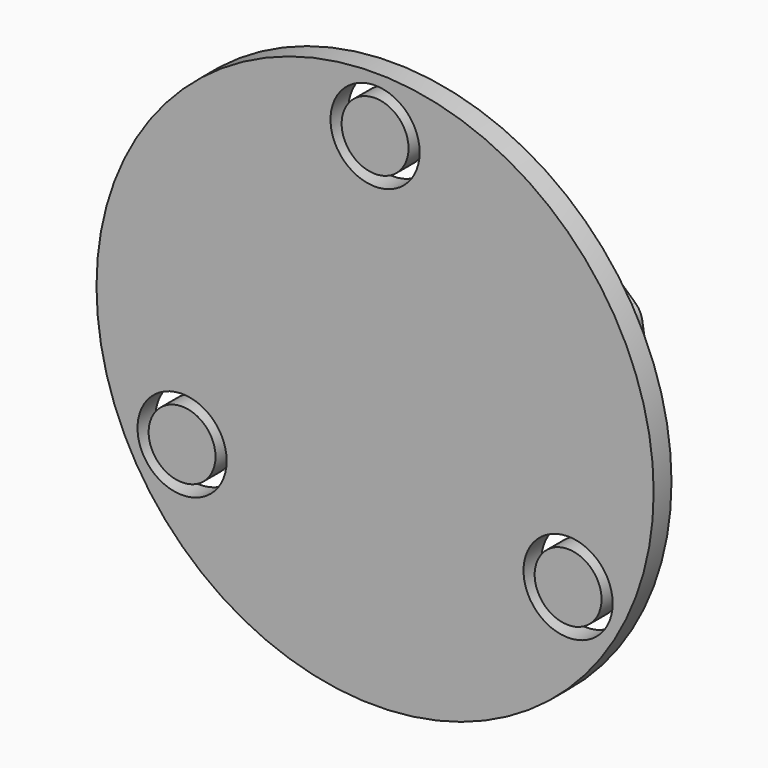
from build123d import *

# Parameters (mm, degrees)
F1_DEPTH      = 13
F2_R          = 1.3
F3_DEPTH      = 5
F4_R          = 1.3
F5_DEPTH      = 25
F6_R          = 1.3
F7_DEPTH      = 5
F8_R          = 25
F9_DEPTH      = 2
F10_R         = 4
F10_R_2       = 3
F11_DEPTH     = 80
F12_T1_DEPTH  = 16.002243982
F12_T3_DEPTH  = 14.8598729542
F12_T5_DEPTH  = 14.7613040686
F12_T7_DEPTH  = 15.2887647241
F12_T9_DEPTH  = 14.7419723435
F12_T11_DEPTH = 14.2482473807


# Not quite as in the source:
# - a fillet or chamfer that OpenCascade refuses, or shapes differently, is made with other operations: its cross-section is extruded or revolved along the edge and cut away or added


with BuildPart() as f1:
    # F0 (on Front) → F1 (new body)
    with BuildSketch(Plane.XZ):
        Polygon((-3.34402165, -12.0443978349), (12.5, 0), (11.86, 3.9484680574), (3.9804532583, 11.1376835822), (-1.1429031284, 12.44764124), (-11.2779609495, 5.390509885), (-12.4032698364, 1.552062294), (-6.9773613512, -10.3714236522), align=None)
    extrude(amount=F1_DEPTH)

    # F2 (on face) → F3 (cut)
    with BuildSketch(Plane(origin=(12.18, 0, 1.9742340287), x_dir=(0, 1, 0), z_dir=(0.9871170143, 0, 0.16))):
        with Locations((-3, 0)):
            Circle(F2_R)
    extrude(amount=-F3_DEPTH, mode=Mode.SUBTRACT)

    # F4 (on face) → F5 (cut)
    with BuildSketch(Plane(origin=(2.9172291114, 0, 11.4095324461), x_dir=(0.9688330447, 0, -0.2477146172), z_dir=(0.2477146172, 0, 0.9688330447))):
        with Locations((-2.1907450021, -3)):
            Circle(F4_R)
    extrude(amount=-F5_DEPTH, mode=Mode.SUBTRACT)

    # F6 (on face) → F7 (cut)
    with BuildSketch(Plane(origin=(-11.840615393, 0, 3.4712860895), x_dir=(0, -1, 0), z_dir=(-0.9596118978, 0, 0.2813272217))):
        with Locations((3, 0)):
            Circle(F6_R)
    extrude(amount=-F7_DEPTH, mode=Mode.SUBTRACT)

    # F8 (on face) → F9 (join)
    with BuildSketch(Plane.XZ.offset(13)):
        Circle(F8_R)
    extrude(amount=F9_DEPTH)

    # F10 (on face) → F11 (cut)
    with BuildSketch(Plane.XZ.offset(15)):
        with Locations((0, 20)):
            Circle(F10_R)
        with Locations((0, 20)):
            Circle(F10_R_2, mode=Mode.SUBTRACT)
        with Locations((17.3205080757, -10)):
            Circle(F10_R)
        with Locations((17.3205080757, -10)):
            Circle(F10_R_2, mode=Mode.SUBTRACT)
        with Locations((-17.3205080757, -10)):
            Circle(F10_R)
        with Locations((-17.3205080757, -10)):
            Circle(F10_R_2, mode=Mode.SUBTRACT)
    extrude(amount=-F11_DEPTH, mode=Mode.SUBTRACT)

    # F12: fillet of radius 2 on 8 edges, made by hand

    # F12_s2 → F12_t1 (cut)
    with BuildSketch(Plane.XZ.offset(-3.002243982)):
        with BuildLine():
            ThreePointArc((-4.4348388753, -11.5421301677), (-3.3803086774, -11.7135390891), (-2.3879978952, -11.3176422991))
            Line((-2.3879978952, -11.3176422991), (-3.34402165, -12.0443978349))
            Line((-3.34402165, -12.0443978349), (-4.4348388753, -11.5421301677))
        make_face()
        with BuildLine():
            ThreePointArc((11.5439762452, -0.7267555357), (12.1909080195, 0.1234763362), (12.3078563852, 1.1854264463))
            Line((12.3078563852, 1.1854264463), (12.5, 0))
            Line((12.5, 0), (11.5439762452, -0.7267555357))
        make_face()
    extrude(amount=F12_T1_DEPTH, mode=Mode.SUBTRACT)

    # F12_s4 → F12_t3 (cut)
    with BuildSketch(Plane.XZ.offset(-1.8598729542)):
        with BuildLine():
            ThreePointArc((-7.2854987693, -9.69428872), (-6.8824804468, -10.2769646373), (-6.3016063269, -10.6825755958))
            Line((-6.3016063269, -10.6825755958), (-6.9773613512, -10.3714236522))
            Line((-6.9773613512, -10.3714236522), (-7.2854987693, -9.69428872))
        make_face()
        with BuildLine():
            ThreePointArc((-12.0951324183, 0.8749273617), (-12.2697226938, 1.5615518796), (-12.1939766801, 2.26596478))
            Line((-12.1939766801, 2.26596478), (-12.4032698364, 1.552062294))
            Line((-12.4032698364, 1.552062294), (-12.0951324183, 0.8749273617))
        make_face()
    extrude(amount=F12_T3_DEPTH, mode=Mode.SUBTRACT)

    # F12_s6 → F12_t5 (cut)
    with BuildSketch(Plane.XZ.offset(-1.7613040686)):
        with BuildLine():
            ThreePointArc((-11.4761620616, 4.7144425491), (-11.1801923355, 5.320140033), (-10.6997935463, 5.793093016))
            Line((-10.6997935463, 5.793093016), (-11.2779609495, 5.390509885))
            Line((-11.2779609495, 5.390509885), (-11.4761620616, 4.7144425491))
        make_face()
    extrude(amount=F12_T5_DEPTH, mode=Mode.SUBTRACT)

    # F12_s8 → F12_t7 (cut)
    with BuildSketch(Plane.XZ.offset(-2.2887647241)):
        with BuildLine():
            ThreePointArc((-1.8942152844, 11.92449587), (-1.1073763077, 12.2512489852), (-0.2559307699, 12.220857049))
            Line((-0.2559307699, 12.220857049), (-1.1429031284, 12.44764124))
            Line((-1.1429031284, 12.44764124), (-1.8942152844, 11.92449587))
        make_face()
    extrude(amount=F12_T7_DEPTH, mode=Mode.SUBTRACT)

    # F12_s10 → F12_t9 (cut)
    with BuildSketch(Plane.XZ.offset(-1.7419723435)):
        with BuildLine():
            ThreePointArc((11.97148623, 3.2606558419), (11.7563010761, 3.8923632844), (11.345263885, 4.4181078717))
            Line((11.345263885, 4.4181078717), (11.86, 3.9484680574))
            Line((11.86, 3.9484680574), (11.97148623, 3.2606558419))
        make_face()
    extrude(amount=F12_T9_DEPTH, mode=Mode.SUBTRACT)

    # F12_s12 → F12_t11 (cut)
    with BuildSketch(Plane.XZ.offset(-1.2482473807)):
        with BuildLine():
            ThreePointArc((3.4967159342, 11.261367231), (3.9512960944, 11.0836676613), (4.3492983836, 10.8011531715))
            Line((4.3492983836, 10.8011531715), (3.9804532583, 11.1376835822))
            Line((3.9804532583, 11.1376835822), (3.4967159342, 11.261367231))
        make_face()
    extrude(amount=F12_T11_DEPTH, mode=Mode.SUBTRACT)


solid = f1.part
